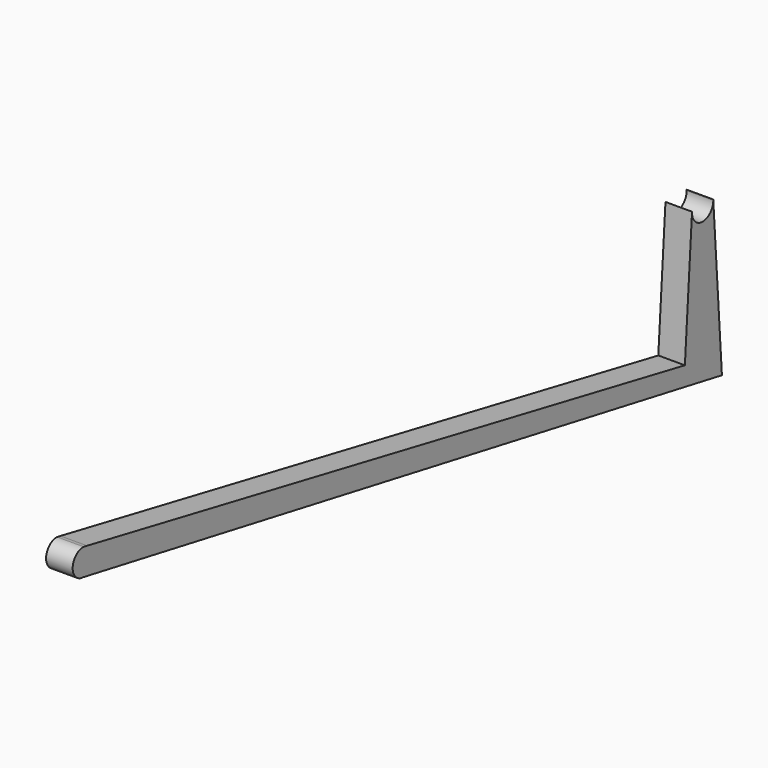
from build123d import *

# Parameters (mm, degrees)
F1_DEPTH = 1.5875


# Not quite as in the source:
# - a feature names something its author has since deleted; it is built from what else it names


with BuildPart() as f1:
    # F0 (on Right) → F1 (new body)
    with BuildSketch(Plane.YZ):
        with BuildLine():
            ThreePointArc((-22.32025, 0.0538603849), (-22.5590646592, -0.5136656763), (-23.1318048474, -0.739689897))
            Line((-23.1318048474, -0.739689897), (24.5522451458, -9.5030463267))
            Line((24.5522451458, -9.5030463267), (23.9059205272, 0))
            ThreePointArc((23.9059205272, 0), (23.9072925, -0.0269146615), (23.90775, -0.0538603849))
            ThreePointArc((23.90775, -0.0538603849), (23.0870542766, -0.8471528848), (22.3220794728, 0))
            Line((22.3220794728, 0), (21.7877844548, -7.8558516301))
            Line((21.7877844548, -7.8558516301), (-22.8339183638, 0.796553686))
            ThreePointArc((-22.8339183638, 0.796553686), (-22.461177719, 0.5053713282), (-22.32025, 0.0538603849))
        make_face()
        with BuildLine():
            Line((-23.0961951526, 0.8474106668), (-23.1318048474, -0.739689897))
            ThreePointArc((-23.1318048474, -0.739689897), (-22.5590646592, -0.5136656763), (-22.32025, 0.0538603849))
            ThreePointArc((-22.32025, 0.0538603849), (-22.461177719, 0.5053713282), (-22.8339183638, 0.796553686))
            Line((-22.8339183638, 0.796553686), (-23.0961951526, 0.8474106668))
        make_face()
        with BuildLine():
            ThreePointArc((-23.0961951526, 0.8474106668), (-23.9075502819, 0.0716652323), (-23.1318048474, -0.739689897))
            Line((-23.1318048474, -0.739689897), (-23.0961951526, 0.8474106668))
        make_face()
    extrude(amount=F1_DEPTH)


solid = f1.part
